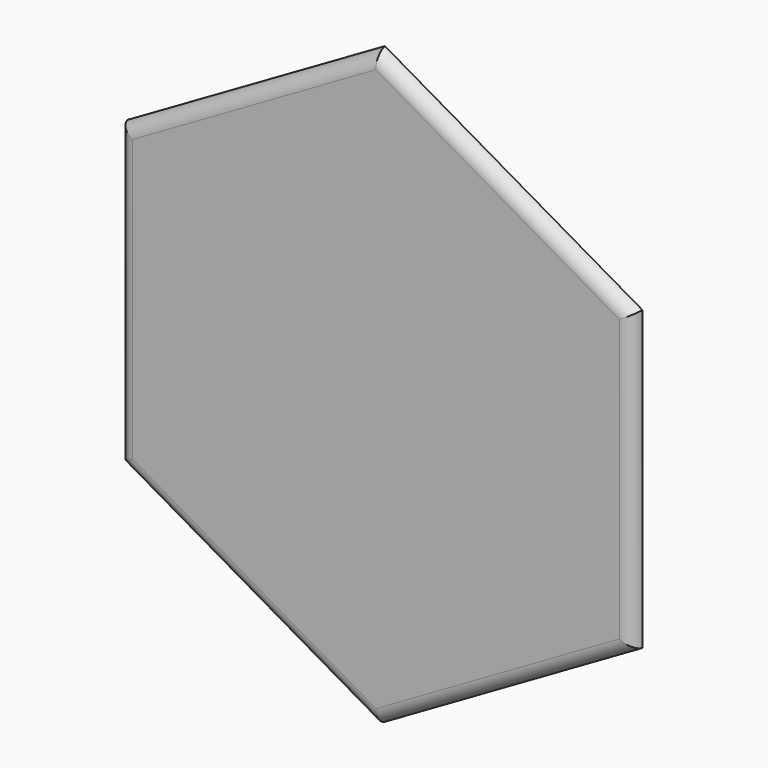
from build123d import *

# Parameters (mm, degrees)
F1_DEPTH     = 4
F2_T1_DEPTH  = 128.417945882
F2_T3_DEPTH  = 128.417945882
F2_T5_DEPTH  = 128.417945882
F2_T7_DEPTH  = 128.417945882
F2_T9_DEPTH  = 128.417945882
F2_T11_DEPTH = 128.417945882


# Not quite as in the source:
# - a fillet or chamfer that OpenCascade refuses, or shapes differently, is made with other operations: its cross-section is extruded or revolved along the edge and cut away or added


with BuildPart() as f1:
    # F0 (on Front) → F1 (new body)
    with BuildSketch(Plane.XZ):
        Polygon((89.9928545723, 51.9738985062), (-0.0142891539, 103.9230474718), (-90.0071437262, 51.9491489656), (-89.9928545723, -51.9738985062), (0.0142891539, -103.9230474718), (90.0071437262, -51.9491489656), align=None)
    extrude(amount=F1_DEPTH)

    # F2: fillet of radius 5 on 6 edges, made by hand

    # F2_s2 → F2_t1 (cut)
    with BuildSketch(Plane(origin=(-0.0088285699, 0, 64.208972334), x_dir=(0, 1, 0), z_dir=(0.0001374974, 0, -0.9999999905))):
        with BuildLine():
            ThreePointArc((0, -90), (-2.8729833462, -88.2632981746), (-4, -85.1010205144))
            Line((-4, -85.1010205144), (-4, -90))
            Line((-4, -90), (0, -90))
        make_face()
    extrude(amount=F2_T1_DEPTH, mode=Mode.SUBTRACT)

    # F2_s4 → F2_t3 (cut)
    with BuildSketch(Plane(origin=(55.6021869072, 0, 32.1121319328), x_dir=(0, 1, 0), z_dir=(-0.8659566469, 0, -0.5001190716))):
        with BuildLine():
            ThreePointArc((0, -90), (-2.8729833462, -88.2632981746), (-4, -85.1010205144))
            Line((-4, -85.1010205144), (-4, -90))
            Line((-4, -90), (0, -90))
        make_face()
    extrude(amount=F2_T3_DEPTH, mode=Mode.SUBTRACT)

    # F2_s6 → F2_t5 (cut)
    with BuildSketch(Plane(origin=(55.6110154771, 0, -32.0968404012), x_dir=(0, 1, 0), z_dir=(-0.8660941443, 0, 0.499880919))):
        with BuildLine():
            ThreePointArc((0, -90), (-2.8729833462, -88.2632981746), (-4, -85.1010205144))
            Line((-4, -85.1010205144), (-4, -90))
            Line((-4, -90), (0, -90))
        make_face()
    extrude(amount=F2_T5_DEPTH, mode=Mode.SUBTRACT)

    # F2_s8 → F2_t7 (cut)
    with BuildSketch(Plane(origin=(0.0088285699, 0, -64.208972334), x_dir=(0, 1, 0), z_dir=(-0.0001374974, 0, 0.9999999905))):
        with BuildLine():
            ThreePointArc((0, -90), (-2.8729833462, -88.2632981746), (-4, -85.1010205144))
            Line((-4, -85.1010205144), (-4, -90))
            Line((-4, -90), (0, -90))
        make_face()
    extrude(amount=F2_T7_DEPTH, mode=Mode.SUBTRACT)

    # F2_s10 → F2_t9 (cut)
    with BuildSketch(Plane(origin=(-55.6021869072, 0, -32.1121319328), x_dir=(0, 1, 0), z_dir=(0.8659566469, 0, 0.5001190716))):
        with BuildLine():
            ThreePointArc((0, -90), (-2.8729833462, -88.2632981746), (-4, -85.1010205144))
            Line((-4, -85.1010205144), (-4, -90))
            Line((-4, -90), (0, -90))
        make_face()
    extrude(amount=F2_T9_DEPTH, mode=Mode.SUBTRACT)

    # F2_s12 → F2_t11 (cut)
    with BuildSketch(Plane(origin=(-55.6110154771, 0, 32.0968404012), x_dir=(0, 1, 0), z_dir=(0.8660941443, 0, -0.499880919))):
        with BuildLine():
            ThreePointArc((0, -90), (-2.8729833462, -88.2632981746), (-4, -85.1010205144))
            Line((-4, -85.1010205144), (-4, -90))
            Line((-4, -90), (0, -90))
        make_face()
    extrude(amount=F2_T11_DEPTH, mode=Mode.SUBTRACT)


solid = f1.part
